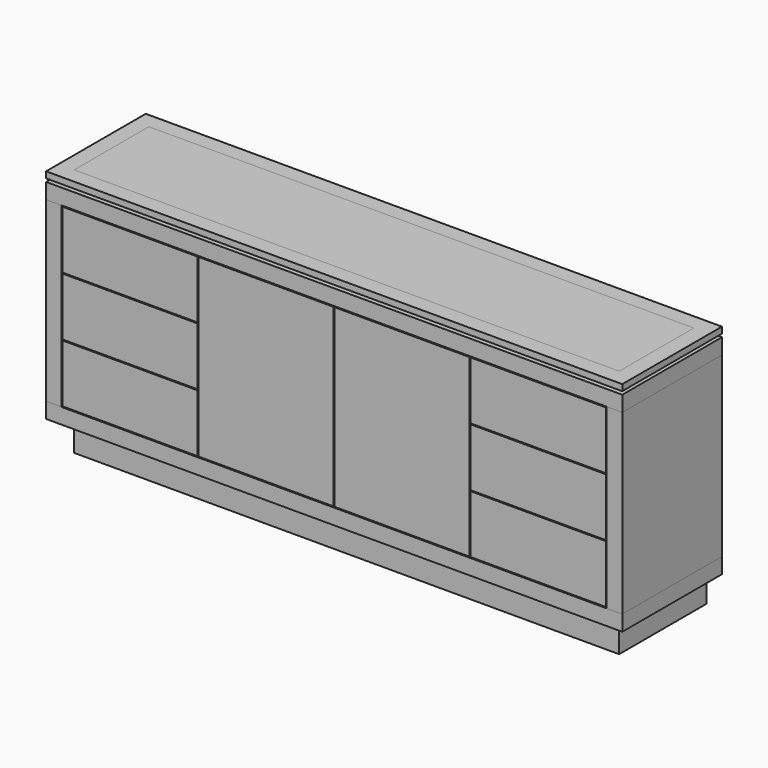
from build123d import *

# Parameters (mm, degrees)
F1_DEPTH  = 400
F0_W      = 50
F0_H      = 50
F0_W_2    = 1750
F0_H_2    = 570
F2_DEPTH  = 400
F3_START  = -50
F0_H_3    = 100
F3_DEPTH  = 350
F0_W_3    = 433.75
F0_H_4    = 186
F4_DEPTH  = 18
F0_H_5    = 3
F5_START  = -20
F5_DEPTH  = 360
F6_DEPTH  = 400
F9_W      = 1750
F9_H      = 300
F10_DEPTH = 5
F11_DEPTH = 3
F12_DEPTH = 2


# Not quite as in the source:
# - a feature names something its author has since deleted; it is built from what else it names


with BuildPart() as f1:
    # F0 (on Front) → F1 (new body)
    with BuildSketch(Plane.XZ):
        Polygon((905, 770), (-875, 770), (-875, 720), (-872, 720), (875, 720), (925, 720), (925, 770), align=None)
        Polygon((-905, 770), (-925, 770), (-925, 720), (-875, 720), (-875, 770), align=None)
    extrude(amount=-F1_DEPTH)


with BuildPart() as f1b:
    # F0 (on Front) → F1, piece 2 (new body)
    with BuildSketch(Plane.XZ):
        with Locations((-900, 125)):
            Rectangle(F0_W, F0_H)
        with Locations((0, 125)):
            Rectangle(F0_W_2, F0_H)
        with Locations((900, 125)):
            Rectangle(F0_W, F0_H)
    extrude(amount=-F1_DEPTH)


with BuildPart() as f2:
    # F0 (on Front) → F2 (new body)
    with BuildSketch(Plane.XZ):
        with Locations((-900, 435)):
            Rectangle(F0_W, F0_H_2)
    extrude(amount=-F2_DEPTH)


with BuildPart() as f2b:
    # F0 (on Front) → F2, piece 2 (new body)
    with BuildSketch(Plane.XZ):
        with Locations((900, 435)):
            Rectangle(F0_W, F0_H_2)
    extrude(amount=-F2_DEPTH)


with BuildPart() as f3:
    # F0 (on Front) → F3 (new body)
    with BuildSketch(Plane.XZ.offset(F3_START)):
        with Locations((0, 50)):
            Rectangle(F0_W_2, F0_H_3)
    extrude(amount=-F3_DEPTH)


with BuildPart() as f4:
    # F0 (on Front) → F4 (new body)
    with BuildSketch(Plane.XZ):
        with Locations((-655.125, 435)):
            Rectangle(F0_W_3, F0_H_4)
    extrude(amount=-F4_DEPTH)


with BuildPart() as f4b:
    # F0 (on Front) → F4, piece 2 (new body)
    with BuildSketch(Plane.XZ):
        with Locations((-655.125, 246)):
            Rectangle(F0_W_3, F0_H_4)
    extrude(amount=-F4_DEPTH)


with BuildPart() as f4c:
    # F0 (on Front) → F4, piece 3 (new body)
    with BuildSketch(Plane.XZ):
        with Locations((-218.375, 435)):
            Rectangle(F0_W_3, F0_H_4)
        with Locations((-218.375, 246)):
            Rectangle(F0_W_3, F0_H_4)
        with Locations((-218.375, 340.5)):
            Rectangle(F0_W_3, F0_H_5)
        with Locations((-218.375, 624)):
            Rectangle(F0_W_3, F0_H_4)
        with Locations((-218.375, 529.5)):
            Rectangle(F0_W_3, F0_H_5)
    extrude(amount=-F4_DEPTH)


with BuildPart() as f4d:
    # F0 (on Front) → F4, piece 4 (new body)
    with BuildSketch(Plane.XZ):
        with Locations((-655.125, 624)):
            Rectangle(F0_W_3, F0_H_4)
    extrude(amount=-F4_DEPTH)


with BuildPart() as f5:
    # F0 (on Front) → F5 (new body)
    with BuildSketch(Plane.XZ.offset(F5_START)):
        Polygon((-905, 780), (-905, 770), (-875, 770), (905, 770), (905, 780), align=None)
    extrude(amount=-F5_DEPTH)


with BuildPart() as f6:
    # F0 (on Front) → F6 (new body)
    with BuildSketch(Plane.XZ):
        Polygon((-925, 780), (-905, 780), (905, 780), (925, 780), (925, 800), (-925, 800), align=None)
    extrude(amount=-F6_DEPTH)

    # F9 (on face) → F10 (cut)
    with BuildSketch(Plane.XY.offset(800)):
        with Locations((0, 200)):
            Rectangle(F9_W, F9_H)
    extrude(amount=-F10_DEPTH, mode=Mode.SUBTRACT)


with BuildPart() as f8_1:
    # F8: instance of F4d
    add(f4d.part.mirror(Plane(origin=(0, 9, 435), x_dir=(0, 1, 0), z_dir=(1, 0, 0))))


with BuildPart() as f8_2:
    # F8: instance of F4
    add(f4.part.mirror(Plane(origin=(0, 9, 435), x_dir=(0, 1, 0), z_dir=(1, 0, 0))))


with BuildPart() as f8_3:
    # F8: instance of F4b
    add(f4b.part.mirror(Plane(origin=(0, 9, 435), x_dir=(0, 1, 0), z_dir=(1, 0, 0))))


with BuildPart() as f8_4:
    # F8: instance of F4c
    add(f4c.part.mirror(Plane(origin=(0, 9, 435), x_dir=(0, 1, 0), z_dir=(1, 0, 0))))


with BuildPart() as f11:
    # F11 (new): a face of the model
    f11_faces = [f6.part.faces().sort_by_distance(p)[0] for p in [
        (0, 200, 795),
    ]]
    extrude(f11_faces, amount=F11_DEPTH)


with BuildPart() as f12:
    # F12 (new): a face of the model
    f12_faces = [f11.part.faces().sort_by_distance(p)[0] for p in [
        (0, 200, 798),
    ]]
    extrude(f12_faces, amount=F12_DEPTH)


solid = Compound([f1.part, f1b.part, f2.part, f2b.part, f3.part, f4.part, f4b.part, f4c.part, f4d.part, f5.part, f6.part, f8_1.part, f8_2.part, f8_3.part, f8_4.part, f11.part, f12.part])
